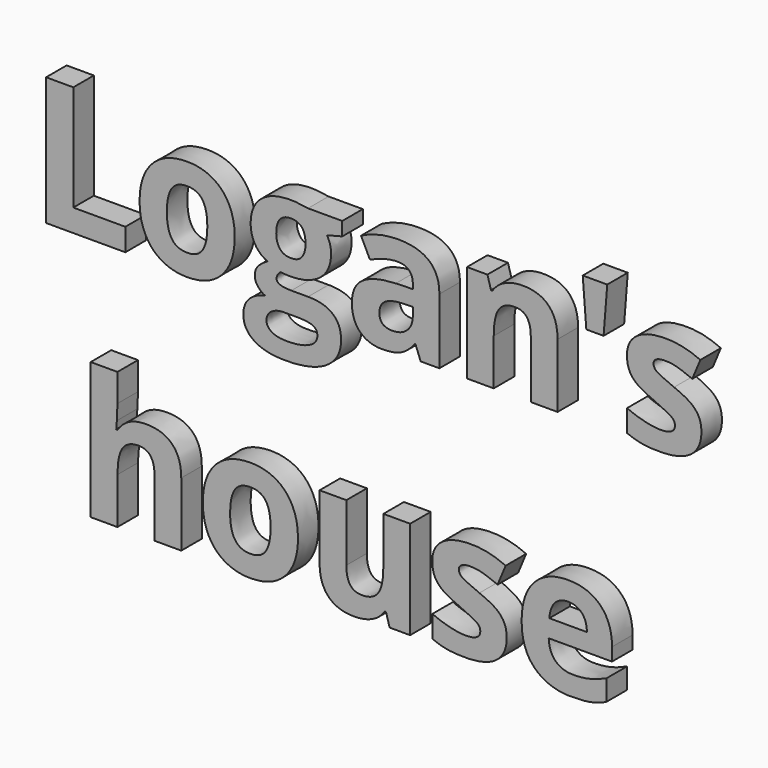
from build123d import *

# Parameters (mm, degrees)
F0_TEXT_SIZE = 74.8927316939
F1_DEPTH     = 10.7


# Not quite as in the source:
# - Text() gives the source's letters only with a copy of the font that has no kerning and outlines rounded to 1/6400 em; it was checked with that copy


with BuildPart() as f1:
    # F0 (on Front) → F1 (new body)
    with BuildSketch(Plane.XZ):
        with Locations((-70.2845528722, 17.3569153994)):
            Text("Logan's", F0_TEXT_SIZE, font='Open Sans', font_style=FontStyle.BOLD, text_align=(TextAlign.LEFT, TextAlign.BOTTOM))
        with Locations((-50.8241446211, -84.4971997042)):
            Text('house', F0_TEXT_SIZE, font='Open Sans', font_style=FontStyle.BOLD, text_align=(TextAlign.LEFT, TextAlign.BOTTOM))
    extrude(amount=F1_DEPTH)


solid = f1.part
